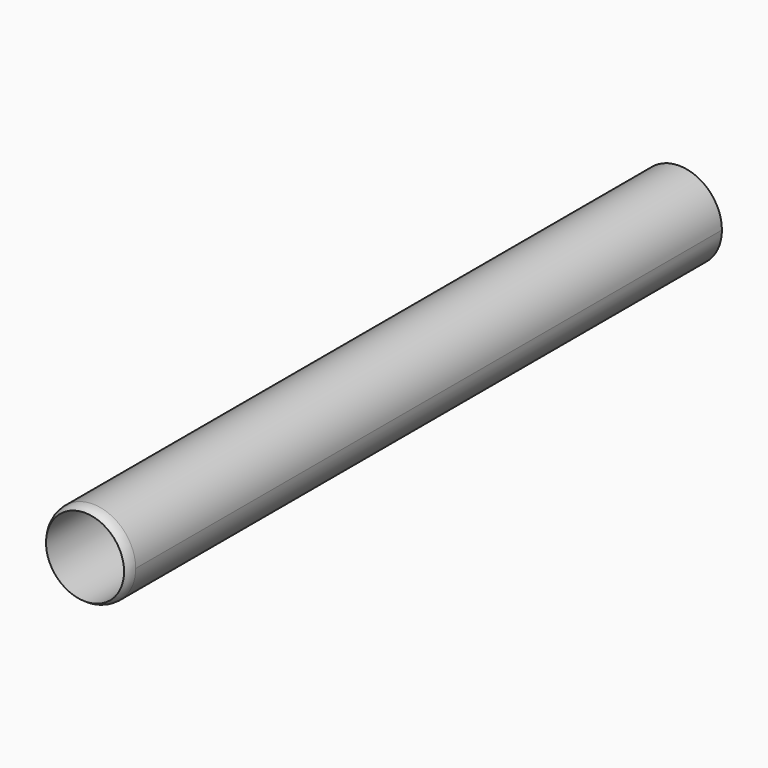
from build123d import *

# Parameters (mm, degrees)
F1_DEPTH = 250


# Not quite as in the source:
# - a fillet or chamfer that OpenCascade refuses, or shapes differently, is made with other operations: its cross-section is extruded or revolved along the edge and cut away or added


with BuildPart() as f1:
    # F0 (on Front) → F1 (new body)
    with BuildSketch(Plane.XZ):
        with BuildLine():
            ThreePointArc((14.3910080635, 0), (-13.3075418668, 5.4781787619), (10.2202866776, -10.1314783379))
            ThreePointArc((10.2202866776, -10.1314783379), (13.3075418668, -5.4781787619), (14.3910080635, 0))
        make_face()
        with BuildLine():
            ThreePointArc((8.400959745, -10.0958666852), (-11.8920367391, 5.5751332681), (13.1340263728, 0))
            ThreePointArc((13.1340263728, 0), (12.3705279138, -4.4127868626), (10.168798903, -8.3125313612))
            ThreePointArc((10.168798903, -8.3125313612), (10.4759385173, -8.7353566894), (10.5845781271, -9.2465449483))
            ThreePointArc((10.5845781271, -9.2465449483), (10.4899428261, -9.7250361614), (10.2202866776, -10.1314783379))
            ThreePointArc((10.2202866776, -10.1314783379), (9.3029968872, -10.5032859052), (8.400959745, -10.0958666852))
        make_face(mode=Mode.SUBTRACT)
        with BuildLine():
            ThreePointArc((10.168798903, -8.3125313612), (9.3275964364, -9.2465449483), (8.400959745, -10.0958666852))
            ThreePointArc((8.400959745, -10.0958666852), (9.3029968872, -10.5032859052), (10.2202866776, -10.1314783379))
            ThreePointArc((10.2202866776, -10.1314783379), (10.4899428261, -9.7250361614), (10.5845781271, -9.2465449483))
            ThreePointArc((10.5845781271, -9.2465449483), (10.4759385173, -8.7353566894), (10.168798903, -8.3125313612))
        make_face()
    extrude(amount=F1_DEPTH)

    # F2: fillet of radius 5 on 1 edges, made by hand

    # F2_s1 → F2_t2 (revolve, cut)
    with BuildSketch(Plane(origin=(0, 0, 0), x_dir=(0, 1, 0), z_dir=(-0.7040144994, 0, -0.7101855987))):
        with BuildLine():
            ThreePointArc((-246.6849111722, 14.3910080635), (-248.4576080518, 14.0662134893), (-250, 13.1340263728))
            Line((-250, 13.1340263728), (-250, 14.3910080635))
            Line((-250, 14.3910080635), (-246.6849111722, 14.3910080635))
        make_face()
    revolve(axis=Axis((0, -250, 0), (0, -1, 0)), mode=Mode.SUBTRACT)


solid = f1.part
